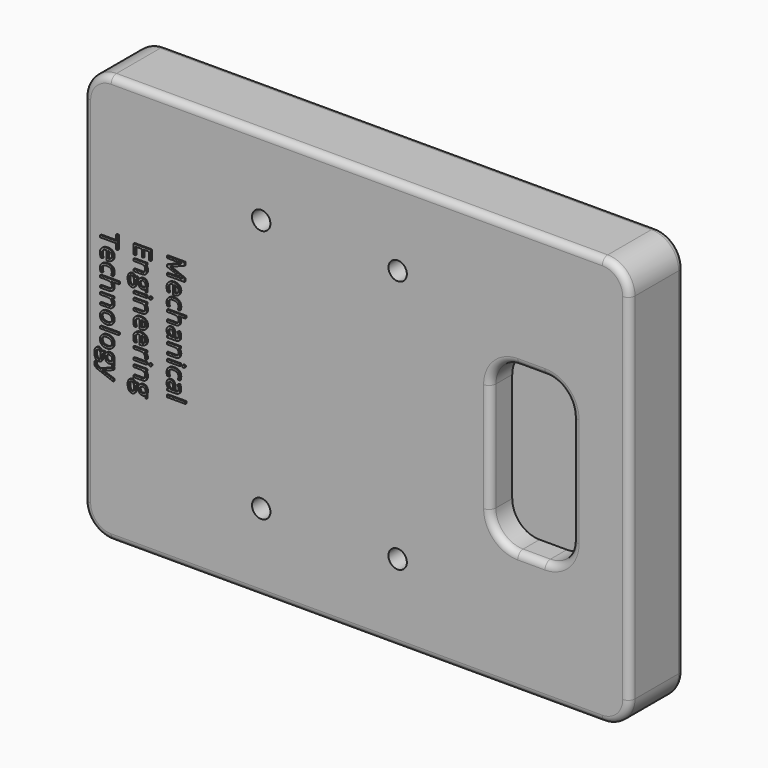
from build123d import *

# Parameters (mm, degrees)
F0_R         = 6.75
F1_DEPTH     = 50
F2_R         = 5
F3_DEPTH     = 30
F4_R         = 13
F4_R_2       = 6.75
F5_DEPTH     = 5
F6_TEXT_SIZE = 17.9523141655
F7_DEPTH     = 1


# Not quite as in the source:
# - Text() gives the source's letters only with a copy of the font that has no kerning and outlines rounded to 1/6400 em; it was checked with that copy


with BuildPart() as f1:
    # F0 (on Front) → F1 (new body)
    with BuildSketch(Plane.XZ):
        with BuildLine():
            ThreePointArc((200, 130), (194.1421356237, 144.1421356237), (180, 150))
            Line((180, 150), (-180, 150))
            ThreePointArc((-180, 150), (-194.1421356237, 144.1421356237), (-200, 130))
            Line((-200, 130), (-200, -130))
            ThreePointArc((-200, -130), (-194.1421356237, -144.1421356237), (-180, -150))
            Line((-180, -150), (180, -150))
            ThreePointArc((180, -150), (194.1421356237, -144.1421356237), (200, -130))
            Line((200, -130), (200, 130))
        make_face()
        with Locations((-70, -93)):
            Circle(F0_R, mode=Mode.SUBTRACT)
        with Locations((30, -93)):
            Circle(F0_R, mode=Mode.SUBTRACT)
        with Locations((-70, 93)):
            Circle(F0_R, mode=Mode.SUBTRACT)
        with BuildLine():
            Line((158, 40), (158, 0))
            Line((158, 0), (158, -40))
            ThreePointArc((158, -40), (152.1421356237, -54.1421356237), (138, -60))
            Line((138, -60), (118, -60))
            ThreePointArc((118, -60), (103.8578643763, -54.1421356237), (98, -40))
            Line((98, -40), (98, 40))
            ThreePointArc((98, 40), (103.8578643763, 54.1421356237), (118, 60))
            Line((118, 60), (138, 60))
            ThreePointArc((138, 60), (152.1421356237, 54.1421356237), (158, 40))
        make_face(mode=Mode.SUBTRACT)
        with Locations((30, 93)):
            Circle(F0_R, mode=Mode.SUBTRACT)
    extrude(amount=F1_DEPTH)

    # F2
    f2_edges = [f1.edges().sort_by_distance(p)[0] for p in [
        (200, 0, 0),
        (200, -50, 0),
        (158, -50, 0),
    ]]
    fillet(f2_edges, radius=F2_R)

    # F0 (on Front) → F3 (join)
    with BuildSketch(Plane.XZ):
        with BuildLine():
            Line((158, -40), (158, 0))
            Line((158, 0), (158, 40))
            ThreePointArc((158, 40), (152.1421356237, 54.1421356237), (138, 60))
            Line((138, 60), (118, 60))
            ThreePointArc((118, 60), (103.8578643763, 54.1421356237), (98, 40))
            Line((98, 40), (98, -40))
            ThreePointArc((98, -40), (103.8578643763, -54.1421356237), (118, -60))
            Line((118, -60), (138, -60))
            ThreePointArc((138, -60), (152.1421356237, -54.1421356237), (158, -40))
        make_face()
    extrude(amount=F3_DEPTH)

    # F4 (on face) → F5 (cut)
    with BuildSketch(Plane.XZ):
        with Locations((30, -93)):
            Circle(F4_R)
        with Locations((30, -93)):
            Circle(F4_R_2, mode=Mode.SUBTRACT)
        with Locations((-70, -93)):
            Circle(F4_R)
        with Locations((-70, -93)):
            Circle(F4_R_2, mode=Mode.SUBTRACT)
        with Locations((-70, 93)):
            Circle(F4_R)
        with Locations((-70, 93)):
            Circle(F4_R_2, mode=Mode.SUBTRACT)
        with Locations((30, 93)):
            Circle(F4_R)
        with Locations((30, 93)):
            Circle(F4_R_2, mode=Mode.SUBTRACT)
    extrude(amount=F5_DEPTH, mode=Mode.SUBTRACT)

    # F6 (on face) → F7 (join)
    with BuildSketch(Plane.XZ.offset(50)):
        with Locations(Location((-138.3817623879, 50), (0, 0, -90))):
            Text('Mechanical', F6_TEXT_SIZE, font='Open Sans', text_align=(TextAlign.LEFT, TextAlign.BOTTOM))
        with Locations(Location((-162.7969096529, 50), (0, 0, -90))):
            Text('Engineering', F6_TEXT_SIZE, font='Open Sans', text_align=(TextAlign.LEFT, TextAlign.BOTTOM))
        with Locations(Location((-187.212056918, 50), (0, 0, -90))):
            Text('Technology', F6_TEXT_SIZE, font='Open Sans', text_align=(TextAlign.LEFT, TextAlign.BOTTOM))
    extrude(amount=F7_DEPTH)


solid = f1.part
